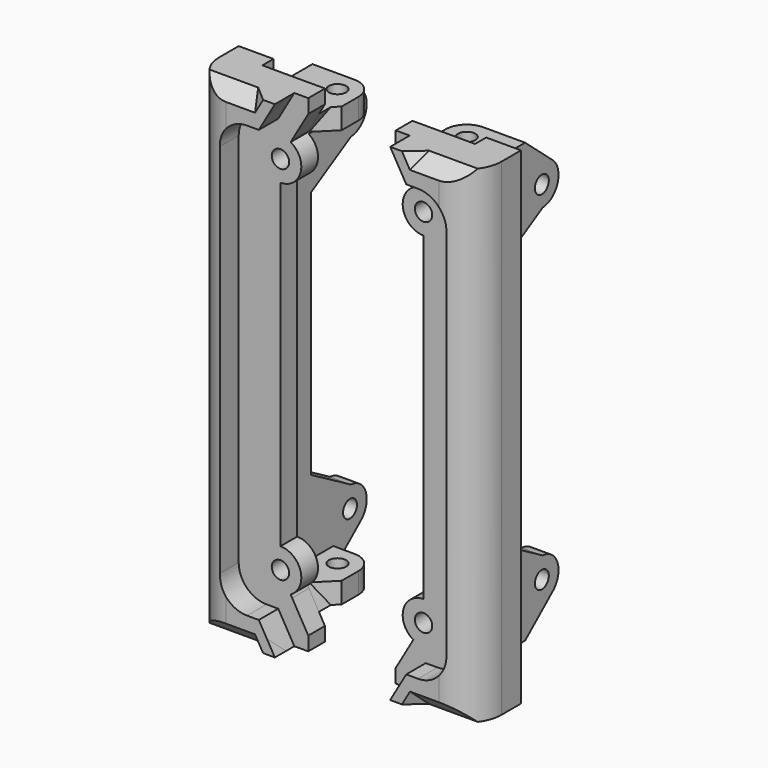
from build123d import *

# Parameters (mm, degrees)
F0_W         = 4
F0_H         = 3
F1_DEPTH     = 6.5
F0_R         = 1.25
F2_DEPTH     = 3
F4_DEPTH     = 8.5
F3_W         = 5
F3_H         = 2
F5_DEPTH     = 12
F7_SIZE      = 2
F8_DEPTH     = 3
F9_SIZE      = 1.99999
F10_R        = 1.25
F11_DEPTH    = 3
F12_T4_DEPTH = 18.4300979278
F12_S5_R     = 3
F12_T6_DEPTH = 11
F13_DEPTH    = 23
F14_R        = 1.25
F15_DEPTH    = 3
F17_T1_DEPTH = 91


# Not quite as in the source:
# - a fillet or chamfer that OpenCascade refuses, or shapes differently, is made with other operations: its cross-section is extruded or revolved along the edge and cut away or added
# - a fillet or chamfer is up to 0.001 mm smaller than in the source, because OpenCascade refuses the exact size


with BuildPart() as f1:
    # F0 (on Front) → F1 (new body)
    with BuildSketch(Plane.XZ):
        Polygon((10.5944581591, 8.801957868), (8.2850570824, 4.801957868), (12.2850570824, 4.801957868), (12.2850570824, 8.801957868), align=None)
        with BuildLine():
            Line((12.2850570824, 8.801957868), (12.2850570824, 4.801957868))
            Line((12.2850570824, 4.801957868), (15.7850570824, 4.801957868))
            Line((15.7850570824, 4.801957868), (20.2850570824, 4.801957868))
            Line((20.2850570824, 4.801957868), (20.2850570824, 9.301957868))
            Line((20.2850570824, 9.301957868), (20.2850570824, 13.801957868))
            Line((20.2850570824, 13.801957868), (16.2850570824, 13.801957868))
            Line((16.2850570824, 13.801957868), (16.2850570824, 12.801957868))
            ThreePointArc((16.2850570824, 12.801957868), (15.1134842071, 9.9735307433), (12.2850570824, 8.801957868))
        make_face()
        with Locations((18.2850570824, 15.301957868)):
            Rectangle(F0_W, F0_H)
    extrude(amount=F1_DEPTH)

    # F0 (on Front) → F2 (join)
    with BuildSketch(Plane.XZ):
        Polygon((10.5944581591, 8.801957868), (8.2850570824, 4.801957868), (12.2850570824, 4.801957868), (12.2850570824, 8.801957868), align=None)
        with BuildLine():
            Line((6.2850570824, 4.801957868), (8.2850570824, 4.801957868))
            Line((8.2850570824, 4.801957868), (10.5944581591, 8.801957868))
            Line((10.5944581591, 8.801957868), (12.2850570824, 8.801957868))
            ThreePointArc((12.2850570824, 8.801957868), (15.1134842071, 9.9735307433), (16.2850570824, 12.801957868))
            Line((16.2850570824, 12.801957868), (16.2850570824, 13.801957868))
            Line((16.2850570824, 13.801957868), (16.2850570824, 16.801957868))
            Line((16.2850570824, 16.801957868), (10.2850570824, 16.801957868))
            ThreePointArc((10.2850570824, 16.801957868), (12.406377426, 15.9232782116), (13.2850570824, 13.801957868))
            ThreePointArc((13.2850570824, 13.801957868), (11.8005749683, 11.2129029174), (8.8162533907, 11.1861184779))
            Line((8.8162533907, 11.1861184779), (8.5944581591, 10.801957868))
            Line((8.5944581591, 10.801957868), (6.2850570824, 6.801957868))
            Line((6.2850570824, 6.801957868), (6.2850570824, 4.801957868))
        make_face()
        with BuildLine():
            Line((12.2850570824, 8.801957868), (12.2850570824, 4.801957868))
            Line((12.2850570824, 4.801957868), (15.7850570824, 4.801957868))
            Line((15.7850570824, 4.801957868), (20.2850570824, 4.801957868))
            Line((20.2850570824, 4.801957868), (20.2850570824, 9.301957868))
            Line((20.2850570824, 9.301957868), (20.2850570824, 13.801957868))
            Line((20.2850570824, 13.801957868), (16.2850570824, 13.801957868))
            Line((16.2850570824, 13.801957868), (16.2850570824, 12.801957868))
            ThreePointArc((16.2850570824, 12.801957868), (15.1134842071, 9.9735307433), (12.2850570824, 8.801957868))
        make_face()
        with Locations((18.2850570824, 15.301957868)):
            Rectangle(F0_W, F0_H)
        with BuildLine():
            ThreePointArc((10.2850570824, 16.801957868), (7.3826857958, 14.5610632064), (8.8162533907, 11.1861184779))
            ThreePointArc((8.8162533907, 11.1861184779), (11.8005749683, 11.2129029174), (13.2850570824, 13.801957868))
            ThreePointArc((13.2850570824, 13.801957868), (12.406377426, 15.9232782116), (10.2850570824, 16.801957868))
        make_face()
        with Locations((10.2850570824, 13.801957868)):
            Circle(F0_R, mode=Mode.SUBTRACT)
    extrude(amount=F2_DEPTH)

    # F3 (on face) → F4 (join)
    with BuildSketch(Plane.XY.offset(16.801957868)):
        Polygon((12.2850570824, 0), (15.2850570824, 0), (15.2850570824, 2), (15.2850570824, 5), (12.2850570824, 5), align=None)
    extrude(amount=-F4_DEPTH)

    # F3 (on face) → F5 (join)
    with BuildSketch(Plane.XY.offset(16.801957868)):
        with Locations((17.7850570824, 1)):
            Rectangle(F3_W, F3_H)
    extrude(amount=-F5_DEPTH)

    # F7
    f7_edges = [f1.edges().sort_by_distance(p)[0] for p in [
        (14.285057, -6.5, 4.801958),
    ]]
    chamfer(f7_edges, length=F7_SIZE)

    # F6 (on face) → F8 (join)
    with BuildSketch(Plane.XZ.offset(6.5)):
        Polygon((9.7850570824, 7.4000340794), (8.2850570824, 4.801957868), (12.2850570824, 4.801957868), (13.7850570824, 7.4000340794), align=None)
    extrude(amount=-F8_DEPTH)

    # F9 (size 2 in the source; OpenCascade refuses exactly that, so slightly less here)
    f9_edges = [f1.edges().sort_by_distance(p)[0] for p in [
        (12.862407, -6.5, 5.801958),
    ]]
    chamfer(f9_edges, length=F9_SIZE)

    # F10 (on face) → F11 (join)
    with BuildSketch(Plane(origin=(0, 0, 8.301957868), x_dir=(1, 0, 0), z_dir=(0, 0, -1))):
        with BuildLine():
            ThreePointArc((9.2850570824, -9), (11.406377426, -8.1213203436), (12.2850570824, -6))
            ThreePointArc((12.2850570824, -6), (9.2850570824, -3), (6.2850570824, -6))
            ThreePointArc((6.2850570824, -6), (7.1637367388, -8.1213203436), (9.2850570824, -9))
        make_face()
        with Locations((9.2850570824, -6)):
            Circle(F10_R, mode=Mode.SUBTRACT)
        with BuildLine():
            ThreePointArc((6.2850570824, -6), (9.2850570824, -3), (12.2850570824, -6))
            ThreePointArc((12.2850570824, -6), (11.406377426, -8.1213203436), (9.2850570824, -9))
            Line((9.2850570824, -9), (15.2850570824, -9))
            Line((15.2850570824, -9), (15.2850570824, -5))
            Line((15.2850570824, -5), (12.2850570824, -5))
            Line((12.2850570824, -5), (12.2850570824, 0))
            Line((12.2850570824, 0), (6.2850570824, 0))
            Line((6.2850570824, 0), (6.2850570824, -6))
        make_face()
    extrude(amount=-F11_DEPTH)

    # F12: chamfer of 3 on 1 edges, made by hand


with BuildPart() as f12_tool2:
    # F12_s3 → F12_t4 (new body)
    with BuildSketch(Plane.XY.offset(0.5869089041)):
        Polygon((6.2850570824, 3), (9.2850570824, 0), (6.2850570824, 0), align=None)
    extrude(amount=F12_T4_DEPTH)

    # F12_s5 → F12_t6 (cut, symmetric)
    with BuildSketch(Plane.XZ.offset(-1.5)):
        with Locations((10.2850570824, 13.801957868)):
            Circle(F12_S5_R)
    extrude(amount=F12_T6_DEPTH, both=True, mode=Mode.SUBTRACT)

    split(bisect_by=Plane(origin=(1.7684586572, 0, -1.0210200818), x_dir=(0, 1, 0), z_dir=(-0.8660254038, 0, 0.5)), keep=Keep.TOP)


with BuildPart() as f1_1:
    add(f1.part)

    # F12_t1: cut F12_tool2
    add(f12_tool2.part, mode=Mode.SUBTRACT)

    # F13 (add): a face of the model
    f13_faces = [f1_1.faces().sort_by_distance(p)[0] for p in [
        (15.9299846186, -0.9275362319, 16.801957868),
    ]]
    extrude(f13_faces, amount=F13_DEPTH)

    # F14 (on face) → F15 (join)
    with BuildSketch(Plane.YZ.offset(15.2850570824)):
        with BuildLine():
            Line((5, 14.801957868), (5, 11.301957868))
            Line((5, 11.301957868), (9, 11.301957868))
            Line((9, 11.301957868), (9, 8.301957868))
            Line((9, 8.301957868), (13.9463414634, 12.5190310388))
            ThreePointArc((13.9463414634, 12.5190310388), (9.1591706072, 13.8377543826), (12.1546210798, 17.7979706053))
            Line((12.1546210798, 17.7979706053), (5, 21.9286930117))
            Line((5, 21.9286930117), (5, 16.801957868))
            Line((5, 16.801957868), (5, 14.801957868))
        make_face()
        with BuildLine():
            ThreePointArc((12.1546210798, 17.7979706053), (9.1591706072, 13.8377543826), (13.9463414634, 12.5190310388))
            ThreePointArc((13.9463414634, 12.5190310388), (14.7238781535, 13.5447833357), (15, 14.801957868))
            ThreePointArc((15, 14.801957868), (14.1753003516, 16.867888259), (12.1546210798, 17.7979706053))
        make_face()
        with Locations((12, 14.801957868)):
            Circle(F14_R, mode=Mode.SUBTRACT)
    extrude(amount=-F15_DEPTH)

    # F16: F1 across face


with BuildPart() as f1_2:
    add(f1_1.part)
    add(f1_1.part.mirror(Plane(origin=(15.9299846186, -0.9275362319, 39.801957868), x_dir=(1, 0, 0), z_dir=(0, 0, 1))))

    # F17: fillet of radius 5 on 1 edges, made by hand

    # F17_s2 → F17_t1 (cut)
    with BuildSketch(Plane.XY.offset(-5.698042132)):
        with BuildLine():
            ThreePointArc((15.2850570824, -6.5), (18.8205909883, -5.0355339059), (20.2850570824, -1.5))
            Line((20.2850570824, -1.5), (20.2850570824, -6.5))
            Line((20.2850570824, -6.5), (15.2850570824, -6.5))
        make_face()
    extrude(amount=F17_T1_DEPTH, mode=Mode.SUBTRACT)


with BuildPart() as f18_1:
    # F18: instance of F1
    add(f1_2.part.mirror(Plane.YZ))


solid = Compound([f1_2.part, f18_1.part])
